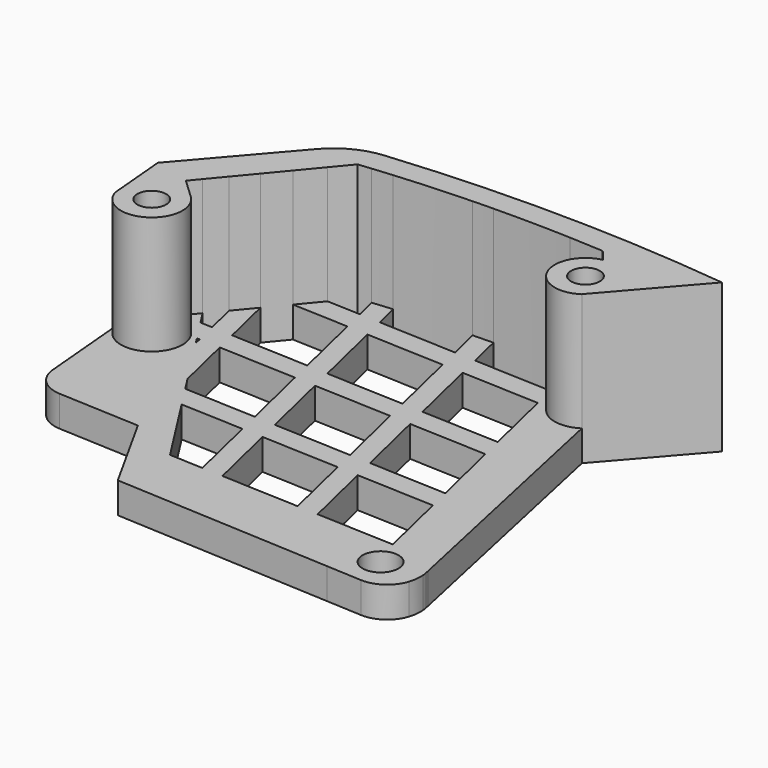
from build123d import *

# Parameters (mm, degrees)
F0_R        = 1.75
F1_DEPTH    = 3
F0_R_2      = 1.4
F2_DEPTH    = 14.5
F3_DEPTH    = 3
F4_R        = 7
F5_T1_DEPTH = 16.6306186867
F5_T3_DEPTH = 4.3681636199
F5_T5_DEPTH = 16.0958411758
F7_DEPTH    = 3


# Not quite as in the source:
# - a fillet or chamfer that OpenCascade refuses, or shapes differently, is made with other operations: its cross-section is extruded or revolved along the edge and cut away or added
# - two fillets or chamfers of one size are made in one step


with BuildPart() as f1:
    # F0 (on Top) → F1 (new body)
    with BuildSketch(Plane.XY):
        with BuildLine():
            Line((-0.4909088138, -1.2505585665), (20.7660850672, -2.35005825))
            Line((20.7660850672, -2.35005825), (25.5381567791, -2.5968895454))
            ThreePointArc((25.5381567791, -2.5968895454), (27.0513379129, -0.9141469555), (27.3799938245, 1.3248986134))
            Line((27.3799938245, 1.3248986134), (27.2720971653, 1.8240689049))
            Line((27.2720971653, 1.8240689049), (21.7261834625, 27.4815394929))
            ThreePointArc((21.7261834625, 27.4815394929), (17.3096816882, 28.8299287619), (19.4503780507, 32.9215128838))
            Line((19.4503780507, 32.9215128838), (18.5115177807, 34.0451927012))
            Line((18.5115177807, 34.0451927012), (15.1742594532, 34.2144082882))
            Line((15.1742594532, 34.2144082882), (15.9797014768, 30.8189948872))
            Line((15.9797014768, 30.8189948872), (16.4916617939, 28.6607800556))
            Line((16.4916617939, 28.6607800556), (18.135858017, 21.7295227758))
            Line((18.135858017, 21.7295227758), (18.644845427, 19.5838405017))
            Line((18.644845427, 19.5838405017), (20.2910235881, 12.6442281836))
            Line((20.2910235881, 12.6442281836), (20.8000109982, 10.4985459094))
            Line((20.8000109982, 10.4985459094), (22.4442072213, 3.5672886297))
            Line((22.4442072213, 3.5672886297), (14.8716080252, 3.8805312748))
            Line((14.8716080252, 3.8805312748), (12.8516365903, 3.9640879479))
            Line((12.8516365903, 3.9640879479), (5.2790373942, 4.2773305929))
            Line((5.2790373942, 4.2773305929), (3.2590659592, 4.360887266))
            Line((3.2590659592, 4.360887266), (0, 4.4956994243))
            Line((0, 4.4956994243), (-4.5071129665, 11.5453820412))
            Line((-4.5071129665, 11.5453820412), (-5.9023623433, 13.727724785))
            Line((-5.9023623433, 13.727724785), (-6.7908302355, 15.1173985523))
            Line((-6.7908302355, 15.1173985523), (-9.9708875905, 20.0914019161))
            Line((-9.9708875905, 20.0914019161), (-10.4149082493, 20.7859051919))
            Line((-10.4149082493, 20.7859051919), (-11.8101576261, 22.9682479357))
            Line((-11.8101576261, 22.9682479357), (-12.6478674294, 24.2785297685))
            Line((-12.6478674294, 24.2785297685), (-13.4783331305, 23.2781674713))
            Line((-13.4783331305, 23.2781674713), (-11.5363753254, 21.4427254814))
            ThreePointArc((-11.5363753254, 21.4427254814), (-12.0316990994, 16.7032264224), (-16.4766345607, 18.4209998989))
            Line((-16.4766345607, 18.4209998989), (-15.4909088138, 7.2494414335))
            Line((-15.4909088138, 7.2494414335), (-4.9353532582, 6.7494414335))
            Line((-4.9353532582, 6.7494414335), (-0.4909088138, -1.2505585665))
        make_face()
        with Locations((23.5090911862, 0.7494414335)):
            Circle(F0_R, mode=Mode.SUBTRACT)
    extrude(amount=F1_DEPTH)

    # F0 (on Top) → F2 (join)
    with BuildSketch(Plane.XY):
        with BuildLine():
            Line((-16.9909088138, 24.2494414335), (-16.4766345607, 18.4209998989))
            ThreePointArc((-16.4766345607, 18.4209998989), (-12.0316990994, 16.7032264224), (-11.5363753254, 21.4427254814))
            Line((-11.5363753254, 21.4427254814), (-13.4783331305, 23.2781674713))
            Line((-13.4783331305, 23.2781674713), (-12.6478674294, 24.2785297685))
            Line((-12.6478674294, 24.2785297685), (-11.3383288336, 25.8559736489))
            Line((-11.3383288336, 25.8559736489), (-9.782692223, 27.729862253))
            Line((-9.782692223, 27.729862253), (-8.1632279798, 29.680636341))
            Line((-8.1632279798, 29.680636341), (-6.4480341787, 31.746724331))
            Line((-6.4480341787, 31.746724331), (-4.9677388347, 33.5298583591))
            ThreePointArc((-4.9677388347, 33.5298583591), (-4.3296328325, 33.596636032), (-3.691225205, 33.6604657178))
            ThreePointArc((-3.691225205, 33.6604657178), (-2.7124843131, 33.7525453098), (-1.7331162834, 33.8376960422))
            ThreePointArc((-1.7331162834, 33.8376960422), (1.9635943301, 34.0963274062), (5.6658885292, 34.2562561568))
            ThreePointArc((5.6658885292, 34.2562561568), (6.6605332405, 34.2823712951), (7.6553394943, 34.3013612736))
            ThreePointArc((7.6553394943, 34.3013612736), (11.4153879508, 34.3087710358), (15.1742594532, 34.2144082882))
            Line((15.1742594532, 34.2144082882), (18.5115177807, 34.0451927012))
            Line((18.5115177807, 34.0451927012), (19.4503780507, 32.9215128838))
            ThreePointArc((19.4503780507, 32.9215128838), (17.3096816882, 28.8299287619), (21.7261834625, 27.4815394929))
            Line((21.7261834625, 27.4815394929), (21.7201782041, 27.5093220636))
            Line((21.7201782041, 27.5093220636), (28.8304557098, 35.6590934098))
            ThreePointArc((28.8304557098, 35.6590934098), (10.8304557098, 36.6599030898), (-7.1695442902, 35.6590934098))
            Line((-7.1695442902, 35.6590934098), (-16.9909088138, 24.2494414335))
        make_face()
        with Locations((-13.5970591864, 19.2624543916)):
            Circle(F0_R_2, mode=Mode.SUBTRACT)
        with Locations((20.077256969, 29.9877400872)):
            Circle(F0_R_2, mode=Mode.SUBTRACT)
    extrude(amount=F2_DEPTH)

    # F0 (on Top) → F3 (join)
    with BuildSketch(Plane.XY):
        with BuildLine():
            Line((-9.782692223, 27.729862253), (-11.3383288336, 25.8559736489))
            Line((-11.3383288336, 25.8559736489), (-10.6418538761, 22.9199207303))
            Line((-10.6418538761, 22.9199207303), (-11.8101576261, 22.9682479357))
            Line((-11.8101576261, 22.9682479357), (-10.4149082493, 20.7859051919))
            Line((-10.4149082493, 20.7859051919), (-10.132866466, 20.7742384561))
            Line((-10.132866466, 20.7742384561), (-9.9708875905, 20.0914019161))
            Line((-9.9708875905, 20.0914019161), (-6.7908302355, 15.1173985523))
            Line((-6.7908302355, 15.1173985523), (-8.112895031, 20.690681783))
            Line((-8.112895031, 20.690681783), (-0.540295835, 20.3774391379))
            Line((-0.540295835, 20.377439138), (1.1058823261, 13.4378268199))
            Line((1.1058823261, 13.4378268199), (-5.9023623433, 13.727724785))
            Line((-5.9023623433, 13.727724785), (-4.5071129665, 11.5453820412))
            Line((-4.5071129665, 11.5453820412), (1.6148697362, 11.2921445457))
            Line((1.6148697362, 11.2921445457), (3.2590659592, 4.360887266))
            Line((3.2590659592, 4.360887266), (5.2790373942, 4.2773305929))
            Line((5.2790373942, 4.2773305929), (3.6348411711, 11.2085878727))
            Line((3.6348411711, 11.2085878727), (11.2074403672, 10.8953452276))
            Line((11.2074403672, 10.8953452276), (12.8516365903, 3.9640879479))
            Line((12.8516365903, 3.9640879479), (14.8716080252, 3.8805312748))
            Line((14.8716080252, 3.8805312748), (13.2274118021, 10.8117885545))
            Line((13.2274118021, 10.8117885545), (20.8000109982, 10.4985459094))
            Line((20.8000109982, 10.4985459094), (20.2910235881, 12.6442281836))
            Line((20.2910235881, 12.6442281836), (12.7184243921, 12.9574708287))
            Line((12.7184243921, 12.9574708287), (11.072246231, 19.8970831467))
            Line((11.072246231, 19.8970831467), (18.644845427, 19.5838405017))
            Line((18.644845427, 19.5838405017), (18.135858017, 21.7295227758))
            Line((18.135858017, 21.7295227758), (10.5632588209, 22.0427654209))
            Line((10.5632588209, 22.0427654209), (8.9190625979, 28.9740227006))
            Line((8.9190625979, 28.9740227006), (16.4916617939, 28.6607800556))
            Line((16.4916617939, 28.6607800556), (15.9797014768, 30.8189948872))
            Line((15.9797014768, 30.8189948872), (8.4071022808, 31.1322375323))
            Line((8.4071022808, 31.1322375323), (7.6553394943, 34.3013612736))
            ThreePointArc((7.6553394943, 34.3013612736), (6.6605332405, 34.2823712951), (5.6658885292, 34.2562561568))
            Line((5.6658885292, 34.2562561568), (6.3871308458, 31.2157942054))
            Line((6.3871308458, 31.2157942054), (-1.1854683502, 31.5290368504))
            Line((-1.1854683502, 31.5290368504), (-1.7331162834, 33.8376960422))
            ThreePointArc((-1.7331162834, 33.8376960422), (-2.7124843131, 33.7525453098), (-3.691225205, 33.6604657178))
            Line((-3.691225205, 33.6604657178), (-3.2054397853, 31.6125935235))
            Line((-3.2054397853, 31.6125935235), (-6.4480341787, 31.746724331))
            Line((-6.4480341787, 31.746724331), (-8.1632279798, 29.680636341))
            Line((-8.1632279798, 29.680636341), (-2.6934794682, 29.4543786918))
            Line((-2.6934794682, 29.4543786918), (-1.0492832451, 22.5231214121))
            Line((-1.0492832451, 22.5231214121), (-8.6218824411, 22.8363640572))
            Line((-8.6218824411, 22.8363640572), (-9.782692223, 27.729862253))
        make_face()
        Polygon((1.4796756, 20.2938824649), (9.052274796, 19.9806398198), (10.6984529571, 13.0410275017), (3.1258537611, 13.3542701468), align=None, mode=Mode.SUBTRACT)
        Polygon((8.543287386, 22.126322094), (0.9706881899, 22.439564739), (-0.6735080331, 29.3708220188), (6.8990911629, 29.0575793737), align=None, mode=Mode.SUBTRACT)
    extrude(amount=F3_DEPTH)

    # F4
    f4_edges = [f1.edges().sort_by_distance(p)[0] for p in [
        (-7.169544, 35.659093, 7.25),
    ]]
    fillet(f4_edges, radius=F4_R)

    # F5: fillet of radius 3 on 3 edges, made by hand

    # F5_s2 → F5_t1 (cut)
    with BuildSketch(Plane.XY.offset(-6.8153093434)):
        with BuildLine():
            ThreePointArc((27.2309502901, -0.4600225022), (26.0778302758, -2.0046934728), (24.2228512202, -2.5288564993))
            Line((24.2228512202, -2.5288564993), (25.5381567791, -2.5968895454))
            ThreePointArc((25.5381567791, -2.5968895454), (26.5766364437, -1.6806211776), (27.2309502901, -0.4600225022))
        make_face()
    extrude(amount=F5_T1_DEPTH, mode=Mode.SUBTRACT)

    # F5_s4 → F5_t3 (cut)
    with BuildSketch(Plane.XY.offset(-0.6840818099)):
        with BuildLine():
            ThreePointArc((27.3520636944, 1.4541138391), (27.3881865873, 1.2545487843), (27.4107435182, 1.0529991394))
            ThreePointArc((27.4107435182, 1.0529991394), (27.3977458408, 1.1892177156), (27.3799938245, 1.3248986134))
            Line((27.3799938245, 1.3248986134), (27.3520636944, 1.4541138391))
        make_face()
    extrude(amount=F5_T3_DEPTH, mode=Mode.SUBTRACT)

    # F5_s6 → F5_t5 (cut)
    with BuildSketch(Plane.XY.offset(-6.5479205879)):
        with BuildLine():
            ThreePointArc((-15.7211174898, 9.8584730948), (-14.8104709381, 7.9581341855), (-12.8746740451, 7.1255145234))
            Line((-12.8746740451, 7.1255145234), (-15.4909088138, 7.2494414335))
            Line((-15.4909088138, 7.2494414335), (-15.7211174898, 9.8584730948))
        make_face()
    extrude(amount=F5_T5_DEPTH, mode=Mode.SUBTRACT)

    # F0 (on Top) → F7 (join)
    with BuildSketch(Plane.XY):
        with Locations((20.077256969, 29.9877400872)):
            Circle(F0_R_2)
        with Locations((-13.5970591864, 19.2624543916)):
            Circle(F0_R_2)
    extrude(amount=F7_DEPTH)


solid = f1.part
